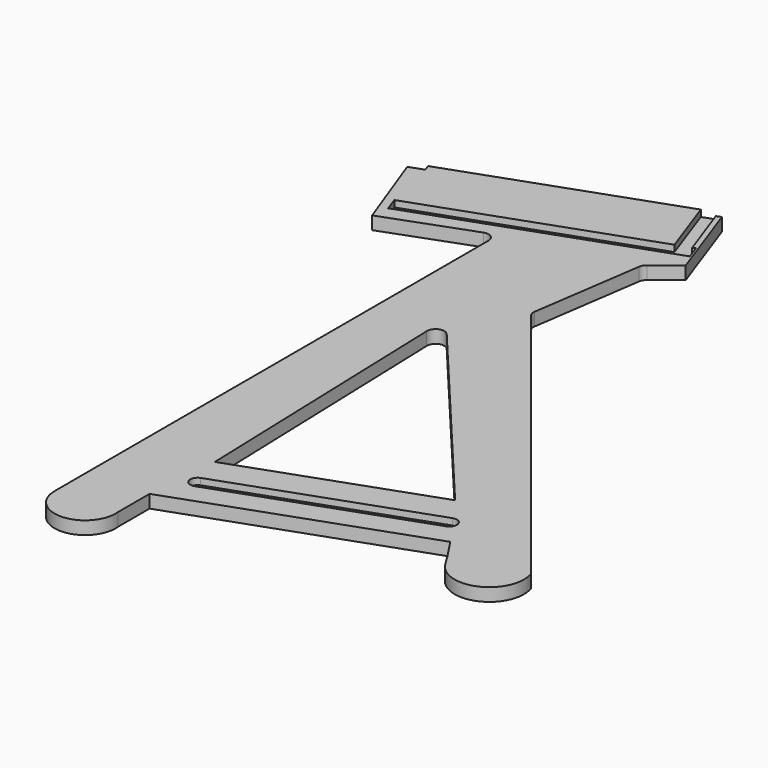
from build123d import *

# Parameters (mm, degrees)
F1_DEPTH = 19.05
F3_DEPTH = 9.525
F5_DEPTH = 9.525


# Not quite as in the source:
# - a feature names something its author has since deleted; it is built from what else it names


with BuildPart() as f1:
    # F0 (on Top) → F1 (new body)
    with BuildSketch(Plane.XY):
        with BuildLine():
            Line((727.2677384075, 427.9083177516), (727.2677384075, -283.5772421425))
            ThreePointArc((727.2677384075, -283.5772421425), (774.3773382982, -328.2348347436), (816.4554812019, -278.8076674308))
            Line((816.4554812019, -278.8076674308), (816.4554812019, -221.0955097314))
            Line((816.4554812019, -221.0955097314), (1159.4623036636, -98.9686407408))
            Line((1159.4623036636, -98.9686407408), (1178.6487772739, -128.0367093729))
            Line((1178.6487772739, -128.0367093729), (1189.3036458742, -145.3996676047))
            ThreePointArc((1189.3036458742, -145.3996676047), (1254.3589120262, -165.180351508), (1280.8355912672, -102.5508970465))
            Line((1280.8355912672, -102.5508970465), (881.2480453078, 396.8848219998))
            ThreePointArc((881.2480453078, 396.8848219998), (878.9075846932, 401.4943033077), (878.5980767553, 406.6546597539))
            Line((878.5980767553, 406.6546597539), (902.2401524871, 568.497452094))
            ThreePointArc((902.2401524871, 568.497452094), (903.8120375637, 573.0182606597), (906.9455405898, 576.6362285378))
            Line((906.9455405898, 576.6362285378), (941.9003890149, 604.1852707886))
            Line((941.9003890149, 604.1852707886), (899.3018677789, 723.8279303566))
            Line((899.3018677789, 723.8279303566), (891.7270738587, 721.1309406639))
            Line((891.7270738587, 721.1309406639), (888.532184766, 730.1041401315))
            Line((888.532184766, 730.1041401315), (557.8398737201, 612.361827435))
            Line((557.8398737201, 612.361827435), (561.0347628128, 603.3886279674))
            Line((561.0347628128, 603.3886279674), (540.3738890749, 596.0323666485))
            Line((540.3738890749, 596.0323666485), (584.2529836062, 476.853404314))
            Line((584.2529836062, 476.853404314), (710.1798289544, 523.2169221936))
            ThreePointArc((710.1798289544, 523.2169221936), (721.8328450807, 521.7157540947), (727.2677384075, 511.2990259602))
            Line((727.2677384075, 511.2990259602), (727.2677384075, 427.9083177516))
        make_face()
        with BuildLine():
            Line((1099.3852571882, -15.0422832395), (825.3589785984, -112.6087723988))
            Line((825.3589785984, -112.6087723988), (812.2279623998, 291.9047427935))
            ThreePointArc((812.2279623998, 291.9047427935), (820.3847868922, 304.1789193457), (834.6503380579, 300.4798321914))
            Line((834.6503380579, 300.4798321914), (1099.3852571882, -15.0422832395))
        make_face(mode=Mode.SUBTRACT)
    extrude(amount=F1_DEPTH)

    # F2 (on face) → F3 (cut)
    with BuildSketch(Plane.XY.offset(19.05)):
        with BuildLine():
            ThreePointArc((837.5686180204, -153.7290348884), (831.0198662622, -167.5195352567), (844.8103666306, -174.068287015))
            Line((844.8103666306, -174.068287015), (1131.9527495937, -71.8318360485))
            ThreePointArc((1131.9527495937, -71.8318360485), (1138.501501352, -58.0413356801), (1124.7110009836, -51.4925839219))
            Line((1124.7110009836, -51.4925839219), (837.5686180204, -153.7290348884))
        make_face()
    extrude(amount=-F3_DEPTH, mode=Mode.SUBTRACT)

    # F4 (on face) → F5 (cut)
    with BuildSketch(Plane.XY.offset(19.05)):
        Polygon((580.3132639661, 522.4942656533), (587.5549912453, 502.1550059319), (931.5862417023, 624.6462138439), (924.4067217173, 644.8107569177), (920.2038128035, 643.3143248671), (892.0960137021, 722.2584502232), (888.9011246094, 731.2316496908), (868.5033081007, 724.1565396792), (899.8030168616, 636.2475531691), align=None)
    extrude(amount=-F5_DEPTH, mode=Mode.SUBTRACT)


solid = f1.part
